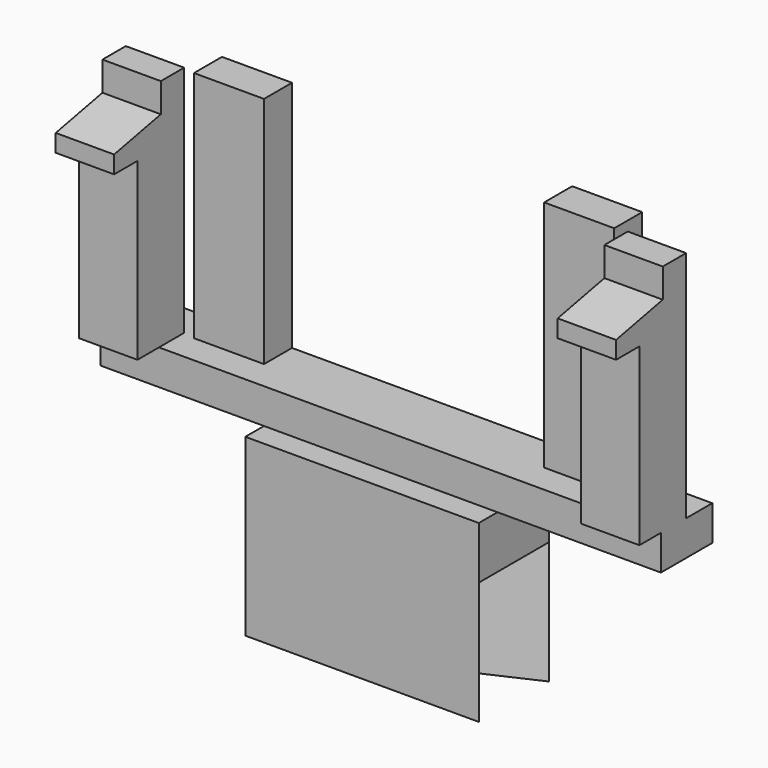
from build123d import *

# Parameters (mm, degrees)
F0_W      = 14
F0_H      = 5.5
F1_DEPTH  = 3
F0_W_2    = 10
F0_H_2    = 2
F2_DEPTH  = 4.5
F4_DEPTH  = 10.5
F5_W      = 6
F5_H      = 3
F5_W_2    = 5
F5_H_2    = 2.7
F5_H_3    = 2.3
F6_DEPTH  = 15
F6_FACE_W = 6
F6_FACE_H = 3
F7_W      = 5
F7_H      = 2.5
F8_DEPTH  = 5
F10_DEPTH = 5
F12_R     = 5


# Not quite as in the source:
# - a feature names something its author has since deleted; it is built from what else it names


with BuildPart() as f1:
    # F0 (on Top) → F1 (new body)
    with BuildSketch(Plane.XY):
        with Locations((17, 0)):
            Rectangle(F0_W, F0_H)
        Polygon((0, -2.75), (10, -2.75), (10, 2.75), (-10, 2.75), (-10, -2.75), align=None)
    extrude(amount=F1_DEPTH)

    # F0 (on Top) → F2 (join)
    with BuildSketch(Plane.XY):
        Polygon((0, -2.75), (10, -2.75), (10, 2.75), (-10, 2.75), (-10, -2.75), align=None)
        with Locations((-5, -3.75)):
            Rectangle(F0_W_2, F0_H_2)
        with Locations((5, -3.75)):
            Rectangle(F0_W_2, F0_H_2)
    extrude(amount=-F2_DEPTH)

    # F3 (on face) → F4 (join)
    with BuildSketch(Plane(origin=(0, 0, -4.5), x_dir=(1, 0, 0), z_dir=(0, 0, -1))):
        Polygon((0, -2.75), (10, -2.75), (4, 0), (0, 0), align=None)
        Polygon((-10, -2.75), (0, -2.75), (0, 0), (-4, 0), align=None)
        Polygon((4, 2), (10, 4.75), (0, 4.75), (0, 2), align=None)
        Polygon((-4, 2), (0, 2), (0, 4.75), (-10, 4.75), align=None)
    extrude(amount=F4_DEPTH)

    # F5 (on face) → F6 (join)
    with BuildSketch(Plane.XY.offset(3)):
        with Locations((15, 1.25)):
            Rectangle(F5_W, F5_H)
        with Locations((21.5, -1.4)):
            Rectangle(F5_W_2, F5_H_2)
        with Locations((21.5, -3.9)):
            Rectangle(F5_W_2, F5_H_3)
    extrude(amount=F6_DEPTH)

    # F6_face (on face) + F7 (on face) → F8 (join)
    with BuildSketch(Plane(origin=(21.5, -2.55, 18), x_dir=(1, 0, 0), z_dir=(0, 0, 1))):
        with Locations((-6.5, 3.8)):
            Rectangle(F6_FACE_W, F6_FACE_H)
    with BuildSketch(Plane.XY.offset(18)):
        with Locations((21.5, -1.3)):
            Rectangle(F7_W, F7_H)
    extrude(amount=F8_DEPTH)

    # F9 (on face) → F10 (join)
    with BuildSketch(Plane.YZ.offset(24)):
        Polygon((-5.05, 18), (-2.55, 18), (-2.55, 19.5), (-7.55, 19.5), (-7.55, 18), align=None)
        Polygon((-7.55, 19.5), (-2.55, 19.5), (-2.55, 20.5), align=None)
    extrude(amount=-F10_DEPTH)

    # F11: F1 across plane


with BuildPart() as f1_1:
    add(f1.part)
    add(f1.part.mirror(Plane.YZ))

    # F12
    f12_edges = [f1_1.edges().sort_by_distance(p)[0] for p in [
        (-4, -2, -9.75),
        (4, -2, -9.75),
        (4, 0, -9.75),
        (-4, 0, -9.75),
    ]]
    fillet(f12_edges, radius=F12_R)


solid = f1_1.part
